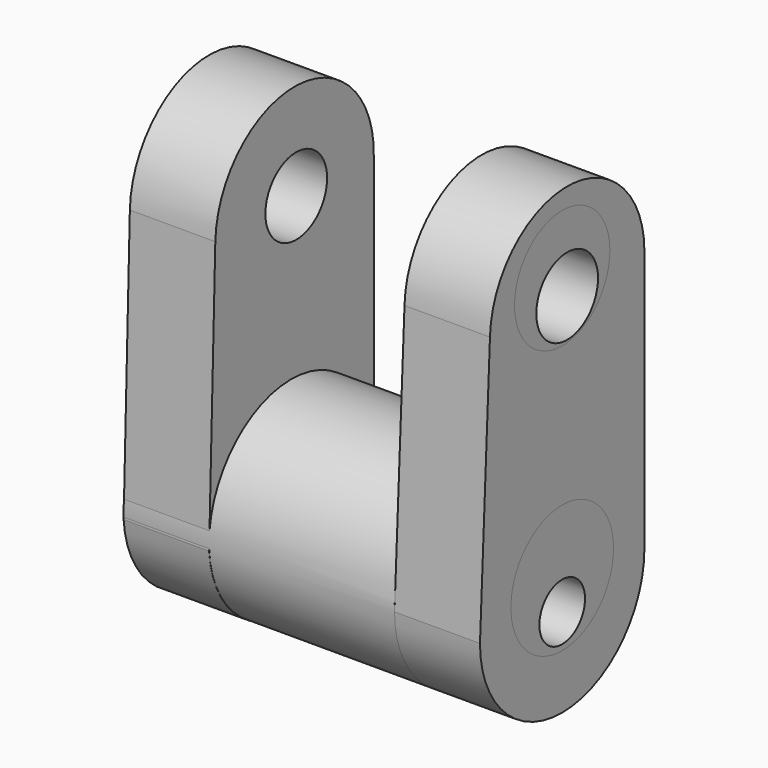
from build123d import *

# Parameters (mm, degrees)
F0_R      = 30.5430762162
F0_R_2    = 21.9615472454
F1_DEPTH  = 80.518
F3_DEPTH  = 25.4
F5_DEPTH  = 25.4
F6_R      = 18.2049933001
F6_R_2    = 16.9331377315
F7_DEPTH  = 24.384
F8_R      = 17.7079617299
F8_R_2    = 19.0588053324
F9_DEPTH  = 24.638
F10_R     = 11.4627485179
F11_DEPTH = 317.246
F12_R     = 8.4753659895
F13_DEPTH = 402.082


# Not quite as in the source:
# - a feature names something its author has since deleted; it is built from what else it names


with BuildPart() as f1:
    # F0 (on Right) → F1 (new body)
    with BuildSketch(Plane.YZ):
        Circle(F0_R)
        Circle(F0_R_2, mode=Mode.SUBTRACT)
    extrude(amount=F1_DEPTH)

    # F2 (on Right) → F3 (join)
    with BuildSketch(Plane.YZ):
        with BuildLine():
            ThreePointArc((-30.5271036923, -2.0653288811), (1.0640567768, -30.6101895865), (30.6584276259, 0))
            Line((30.6584276259, 0), (30.6584276259, 76.3430893421))
            ThreePointArc((30.6584276259, 76.3430893421), (2.0369783495, 106.5633685136), (-28.2157845795, 77.976256609))
            Line((-28.2157845795, 77.976256609), (-30.5271036923, -2.0653288811))
        make_face()
    extrude(amount=F3_DEPTH)

    # F4 (on face) → F5 (join)
    with BuildSketch(Plane.YZ.offset(80.518)):
        with BuildLine():
            Line((-26.8347635865, 78.6278471351), (-30.5430762162, 0))
            ThreePointArc((-30.5430762162, 0), (0, -30.5430762162), (30.5430762162, 0))
            Line((30.5430762162, 0), (30.5430762162, 77.7075961232))
            ThreePointArc((30.5430762162, 77.7075961232), (2.3069613013, 106.4002056349), (-26.8347635865, 78.6278471351))
        make_face()
    extrude(amount=F5_DEPTH)

    # F6 (on Right) → F7 (join)
    with BuildSketch(Plane.YZ):
        Circle(F6_R)
        with Locations((0, 80.0817832351)):
            Circle(F6_R_2)
    extrude(amount=F7_DEPTH)

    # F8 (on face) → F9 (join)
    with BuildSketch(Plane.YZ.offset(105.918)):
        with Locations((0, 83.1589326262)):
            Circle(F8_R)
        with Locations((0, 4.7338949516)):
            Circle(F8_R_2)
    extrude(amount=-F9_DEPTH)

    # F10 (on face) → F11 (cut)
    with BuildSketch(Plane.YZ.offset(105.918)):
        with Locations((1.8467766198, 77.7075961232)):
            Circle(F10_R)
    extrude(amount=-F11_DEPTH, mode=Mode.SUBTRACT)

    # F12 (on face) → F13 (cut)
    with BuildSketch(Plane.YZ.offset(105.918)):
        with Locations((0, -4.1660955176)):
            Circle(F12_R)
    extrude(amount=-F13_DEPTH, mode=Mode.SUBTRACT)


solid = f1.part
